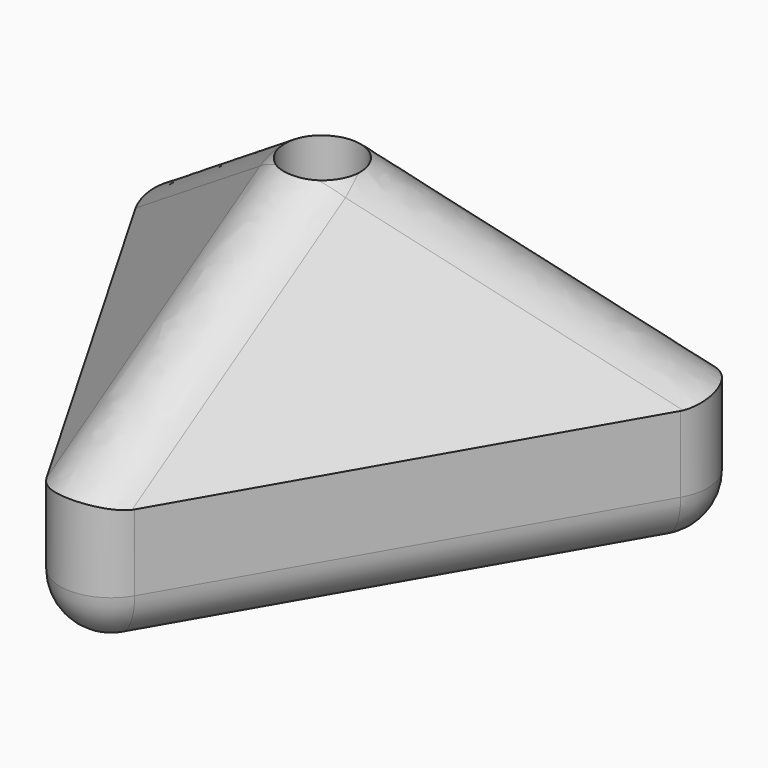
from build123d import *

# Parameters (mm, degrees)
F4_R          = 5
F9_DEPTH      = 10
F10_T1_DEPTH  = 23.3205080757
F10_T3_DEPTH  = 36.1435935394
F10_T5_DEPTH  = 36.1435935394
F10_T7_DEPTH  = 36.1435935394
F10_T12_DEPTH = 4
F10_T18_DEPTH = 4
F10_T24_DEPTH = 4
F6_R          = 2.7
F11_DEPTH     = 8
F8_R          = 3
F12_DEPTH     = 25
F13_R         = 2.5


# Not quite as in the source:
# - a fillet or chamfer that OpenCascade refuses, or shapes differently, is made with other operations: its cross-section is extruded or revolved along the edge and cut away or added


with BuildPart() as f3:
    # F0 (on Top) → F3 section 0
    with BuildSketch(Plane.XY, mode=Mode.PRIVATE) as f3_s0:
        Polygon((25, 14.4337567297), (-25, 14.4337567297), (0, -28.8675134595), align=None)
    loft([f3_s0.sketch, Vertex(0, 0, 18)])

    # F4
    f4_edges = [f3.edges().sort_by_distance(p)[0] for p in [
        (12.5, 7.216878, 9),
        (0, -14.433757, 9),
        (-12.5, 7.216878, 9),
    ]]
    fillet(f4_edges, radius=F4_R)

    # F0 (on Top) → F9 (join)
    with BuildSketch(Plane.XY):
        Polygon((25, 14.4337567297), (-25, 14.4337567297), (0, -28.8675134595), align=None)
    extrude(amount=-F9_DEPTH)

    # F10: fillet of radius 4 on 6 edges, made by hand

    # F10_s2 → F10_t1 (cut)
    with BuildSketch(Plane.XY.offset(-6)):
        with BuildLine():
            ThreePointArc((21.5358983849, 8.4337567297), (21.5358983849, 12.4337567297), (18.0717967697, 14.4337567297))
            Line((18.0717967697, 14.4337567297), (25, 14.4337567297))
            Line((25, 14.4337567297), (21.5358983849, 8.4337567297))
        make_face()
        with BuildLine():
            ThreePointArc((-21.5358983849, 8.4337567297), (-21.5358983849, 12.4337567297), (-18.0717967697, 14.4337567297))
            Line((-18.0717967697, 14.4337567297), (-25, 14.4337567297))
            Line((-25, 14.4337567297), (-21.5358983849, 8.4337567297))
        make_face()
        with BuildLine():
            ThreePointArc((3.4641016151, -22.8675134595), (0, -24.8675134595), (-3.4641016151, -22.8675134595))
            Line((-3.4641016151, -22.8675134595), (0, -28.8675134595))
            Line((0, -28.8675134595), (3.4641016151, -22.8675134595))
        make_face()
    extrude(amount=F10_T1_DEPTH, mode=Mode.SUBTRACT)

    # F10_s4 → F10_t3 (cut)
    with BuildSketch(Plane.YZ.offset(-18.0717967697)):
        with BuildLine():
            ThreePointArc((14.4337567297, -6), (13.2621838545, -8.8284271247), (10.4337567297, -10))
            Line((10.4337567297, -10), (14.4337567297, -10))
            Line((14.4337567297, -10), (14.4337567297, -6))
        make_face()
    extrude(amount=F10_T3_DEPTH, mode=Mode.SUBTRACT)

    # F10_s6 → F10_t5 (cut)
    with BuildSketch(Plane(origin=(-9.0358983849, 15.6506350946, 0), x_dir=(0, 0, 1), z_dir=(0.5, -0.8660254038, 0))):
        with BuildLine():
            ThreePointArc((-6, 14.4337567297), (-8.8284271247, 13.2621838545), (-10, 10.4337567297))
            Line((-10, 10.4337567297), (-10, 14.4337567297))
            Line((-10, 14.4337567297), (-6, 14.4337567297))
        make_face()
    extrude(amount=F10_T5_DEPTH, mode=Mode.SUBTRACT)

    # F10_s8 → F10_t7 (cut)
    with BuildSketch(Plane(origin=(-9.0358983849, -15.6506350946, 0), x_dir=(0, 0, 1), z_dir=(0.5, 0.8660254038, 0))):
        with BuildLine():
            ThreePointArc((-6, 14.4337567297), (-8.8284271247, 13.2621838545), (-10, 10.4337567297))
            Line((-10, 10.4337567297), (-10, 14.4337567297))
            Line((-10, 14.4337567297), (-6, 14.4337567297))
        make_face()
    extrude(amount=F10_T7_DEPTH, mode=Mode.SUBTRACT)


with BuildPart() as f10_tool10:
    # F10_s11 → F10_t12 (new body)
    with BuildSketch(Plane.XY.offset(-6)):
        Polygon((18.0717967697, 10.4337567297), (21.5358983849, 8.4337567297), (25, 14.4337567297), (18.0717967697, 14.4337567297), align=None)
    extrude(amount=-F10_T12_DEPTH)

    # F10_s13 → F10_t14 (revolve, cut)
    with BuildSketch(Plane(origin=(18.0717967697, 10.4337567297, -6), x_dir=(-0.8660254038, -0.5, 0), z_dir=(0.5, -0.8660254038, 0))):
        with BuildLine():
            ThreePointArc((0, -4), (4, 0), (0, 4))
            Line((0, 4), (0, -4))
        make_face()
    revolve(axis=Axis((18.0717967697, 10.4337567297, -6), (0, 0, -1)), mode=Mode.SUBTRACT)


with BuildPart() as f3_1:
    add(f3.part)

    # F10_t9: cut F10_tool10
    add(f10_tool10.part, mode=Mode.SUBTRACT)


with BuildPart() as f10_tool16:
    # F10_s17 → F10_t18 (new body)
    with BuildSketch(Plane.XY.offset(-6)):
        Polygon((-18.0717967697, 10.4337567297), (-21.5358983849, 8.4337567297), (-25, 14.4337567297), (-18.0717967697, 14.4337567297), align=None)
    extrude(amount=-F10_T18_DEPTH)

    # F10_s19 → F10_t20 (revolve, cut)
    with BuildSketch(Plane(origin=(-18.0717967697, 10.4337567297, -6), x_dir=(0.8660254038, -0.5, 0), z_dir=(0.5, 0.8660254038, 0))):
        with BuildLine():
            ThreePointArc((0, -4), (4, 0), (0, 4))
            Line((0, 4), (0, -4))
        make_face()
    revolve(axis=Axis((-18.0717967697, 10.4337567297, -6), (0, 0, -1)), mode=Mode.SUBTRACT)


with BuildPart() as f3_2:
    add(f3_1.part)

    # F10_t15: cut F10_tool16
    add(f10_tool16.part, mode=Mode.SUBTRACT)


with BuildPart() as f10_tool22:
    # F10_s23 → F10_t24 (new body)
    with BuildSketch(Plane.XY.offset(-6)):
        Polygon((0, -20.8675134595), (3.4641016151, -22.8675134595), (0, -28.8675134595), (-3.4641016151, -22.8675134595), align=None)
    extrude(amount=-F10_T24_DEPTH)

    # F10_s25 → F10_t26 (revolve, cut)
    with BuildSketch(Plane(origin=(0, -20.8675134595, -6), x_dir=(0, 1, 0), z_dir=(-1, 0, 0))):
        with BuildLine():
            ThreePointArc((0, -4), (4, 0), (0, 4))
            Line((0, 4), (0, -4))
        make_face()
    revolve(axis=Axis((0, -20.8675134595, -6), (0, 0, -1)), mode=Mode.SUBTRACT)


with BuildPart() as f3_3:
    add(f3_2.part)

    # F10_t21: cut F10_tool22
    add(f10_tool22.part, mode=Mode.SUBTRACT)

    # F6 (on offset) → F11 (cut)
    with BuildSketch(Plane.XY.offset(-9)):
        Circle(F6_R)
    extrude(amount=F11_DEPTH, mode=Mode.SUBTRACT)

    # F8 (on offset) → F12 (cut)
    with BuildSketch(Plane.XY.offset(-1)):
        Circle(F8_R)
    extrude(amount=F12_DEPTH, mode=Mode.SUBTRACT)

    # F13
    f13_edges = [f3_3.edges().sort_by_distance(p)[0] for p in [
        (-2.7, 0, -9),
    ]]
    fillet(f13_edges, radius=F13_R)


solid = f3_3.part
